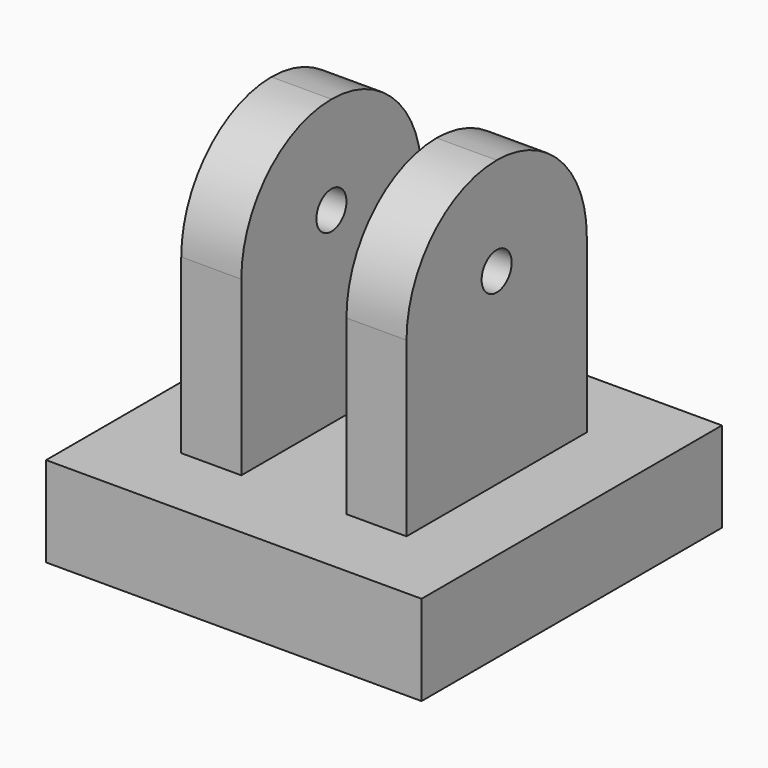
from build123d import *

# Parameters (mm, degrees)
F0_W     = 50
F0_H     = 50
F1_DEPTH = 10
F2_W     = 8
F2_H     = 30
F4_DEPTH = 40
F3_W     = 8
F3_H     = 30
F5_DEPTH = 40
F6_R     = 14.99999
F8_D     = 5
F9_DEPTH = 2


# Not quite as in the source:
# - a fillet or chamfer is up to 0.001 mm smaller than in the source, because OpenCascade refuses the exact size


with BuildPart() as f1:
    # F0 (on Top) → F1 (new body)
    with BuildSketch(Plane.XY):
        with Locations((-3.097159788, 1.3252983437)):
            Rectangle(F0_W, F0_H)
    extrude(amount=F1_DEPTH)

    # F2 (on face) → F4 (join)
    with BuildSketch(Plane.XY.offset(10)):
        with Locations((-14.097159788, 1.3252983437)):
            Rectangle(F2_W, F2_H)
    extrude(amount=F4_DEPTH)

    # F3 (on face) → F5 (join)
    with BuildSketch(Plane.XY.offset(10)):
        with Locations((7.902840212, 1.3252983437)):
            Rectangle(F3_W, F3_H)
    extrude(amount=F5_DEPTH)

    # F6 (radius 15 in the source; OpenCascade refuses exactly that, so slightly less here)
    f6_edges = [f1.edges().sort_by_distance(p)[0] for p in [
        (7.90284, -13.674702, 50),
        (7.90284, 16.325298, 50),
        (-14.09716, -13.674702, 50),
        (-14.09716, 16.325298, 50),
    ]]
    fillet(f6_edges, radius=F6_R)

    # F8 (through all)
    with Locations(Plane(origin=(-18.097159788, 0, 0), x_dir=(0, -1, 0), z_dir=(-1, 0, 0))):
        with Locations((-1.3252983437, 36.9870997965)):
            Hole(F8_D / 2)

    # F9 (add): a face of the model
    f9_faces = [f1.faces().sort_by_distance(p)[0] for p in [
        (-3.097159788, 1.3252983437, 10),
    ]]
    extrude(f9_faces, amount=F9_DEPTH)


solid = f1.part
